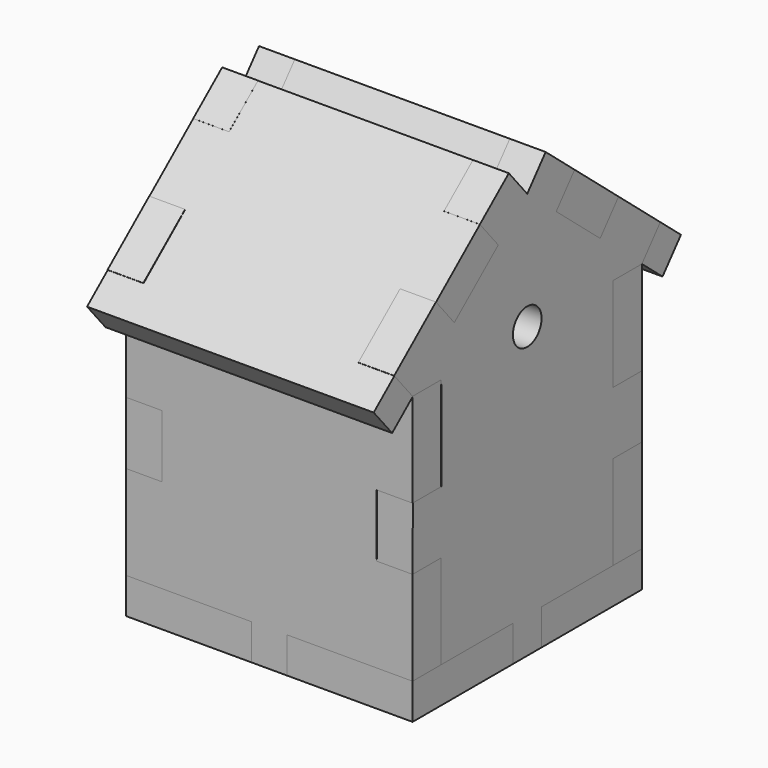
from build123d import *

# Parameters (mm, degrees)
F1_DEPTH  = 12.7
F2_W      = 25.5417573869
F2_H      = 12.7
F3_DEPTH  = 12.7
F4_R      = 6.35
F5_DEPTH  = 12.7
F8_W      = 101.6
F8_H      = 78.1991302645
F9_DEPTH  = 12.7
F10_ANGLE = 180
F11_ANGLE = 80
F15_R     = 3.556
F16_DEPTH = 25.4


with BuildPart() as f1:
    # F0 (on Top) → F1 (new body)
    with BuildSketch(Plane.XY):
        Polygon((-6.35, 50.8), (-50.8, 50.8), (-50.8, 6.35), (-38.1, 6.35), (-38.1, -6.35), (-50.8, -6.35), (-50.8, -50.8), (-6.35, -50.8), (-6.35, -38.1), (6.35, -38.1), (6.35, -50.8), (50.8, -50.8), (50.8, -6.35), (38.1, -6.35), (38.1, 6.35), (50.8, 6.35), (50.8, 50.8), (6.35, 50.8), (6.35, 38.1), (-6.35, 38.1), align=None)
    extrude(amount=F1_DEPTH)


with BuildPart() as f3:
    # F2 (on face) → F3 (new body)
    with BuildSketch(Plane(origin=(0, 50.8, 0), x_dir=(-1, 0, 0), z_dir=(0, 1, 0))):
        Polygon((-6.35, 12.7), (-6.35, 0), (6.35, 0), (6.35, 12.7), (50.8, 12.7), (50.8, 46.0375), (38.1, 46.0375), (38.1, 68.2625), (50.8, 68.2625), (50.8, 101.6), (12.7, 101.6), (12.7, 88.9), (-12.8417573869, 88.9), (-12.8417573869, 101.6), (-50.8, 101.6), (-50.8, 68.2625), (-38.1, 68.2625), (-38.1, 46.0375), (-50.8, 46.0375), (-50.8, 12.7), align=None)
        with Locations((-0.0708786935, 95.25)):
            Rectangle(F2_W, F2_H)
    extrude(amount=-F3_DEPTH)


with BuildPart() as f5:
    # F4 (on face) → F5 (new body)
    with BuildSketch(Plane(origin=(-50.8, 0, 0), x_dir=(0, -1, 0), z_dir=(-1, 0, 0))):
        Polygon((-50.8, 101.6), (-38.1, 101.6), (-38.1, 68.2625), (-50.8, 68.2625), (-50.8, 46.0375), (-38.1, 46.0375), (-38.1, 12.7), (-6.35, 12.7), (-6.35, 0), (6.35, 0), (6.35, 12.7), (38.1, 12.7), (38.1, 46.0375), (50.8, 46.0375), (50.6797134876, 68.2625), (37.9797134876, 68.2625), (38.1, 101.6), (50.8, 101.6), (58.9537135117, 111.336886359), (40.4657224209, 126.8188153046), (32.3120089092, 117.0819289456), (12.8382361911, 133.389355969), (20.9919497028, 143.126242328), (8.1537135117, 153.8770404824), (0, 144.1401541233), (-8.1537135117, 153.8770404824), (-20.9919497028, 143.126242328), (-12.8382361911, 133.389355969), (-32.3120089092, 117.0819289456), (-40.4657224209, 126.8188153046), (-58.9537135117, 111.336886359), align=None)
        with Locations((0, 102.6944294572)):
            Circle(F4_R, mode=Mode.SUBTRACT)
    extrude(amount=-F5_DEPTH)


with BuildPart() as f6_1:
    # F6: copy of F5
    add(f5.part.moved(Location((88.9, 0, 0))))


with BuildPart() as f7_1:
    # F7: copy of F3
    add(f3.part.moved(Location((0, -88.9, 0))))


with BuildPart() as f9:
    # F8 (on face) → F9 (new body)
    with BuildSketch(Plane(origin=(0, 70.9501126824, 84.7262027734), x_dir=(1, 0, 0), z_dir=(0, 0.642024686, 0.7666839653))):
        with Locations((0, -53.4419720532)):
            Rectangle(F8_W, F8_H)
    extrude(amount=F9_DEPTH)


with BuildPart() as f10_1:
    # F10: copy of F9
    add(f9.part.rotate(Axis((-50.8, 4.0768567559, 149.0085973028), (0, 0.642024686, 0.7666839653)), F10_ANGLE))


with BuildPart() as f10_1_1:
    # F11: moved
    add(f10_1.part.rotate(Axis((-101.6, 0, 144.1401541233), (1, 0, 0)), F11_ANGLE))


with BuildPart() as f10_1_2:
    # F12: moved
    add(f10_1_1.part.moved(Location((101.6, 0, 0))))

    # F14: cut F6_1, F5
    add(f6_1.part, mode=Mode.SUBTRACT)
    add(f5.part, mode=Mode.SUBTRACT)


with BuildPart() as f9_1:
    add(f9.part)

    # F13: cut F5
    add(f5.part, mode=Mode.SUBTRACT)

    # F17: cut F6_1
    add(f6_1.part, mode=Mode.SUBTRACT)


with BuildPart() as f5_1:
    add(f5.part)

    # F15 (on face) → F16 (cut)
    with BuildSketch(Plane(origin=(-50.8, 0, 0), x_dir=(0, -1, 0), z_dir=(-1, 0, 0))):
        with Locations((0, 90.3551727533)):
            Circle(F15_R)
    extrude(amount=-F16_DEPTH, mode=Mode.SUBTRACT)


solid = Compound([f1.part, f3.part, f6_1.part, f7_1.part, f10_1_2.part, f9_1.part, f5_1.part])
